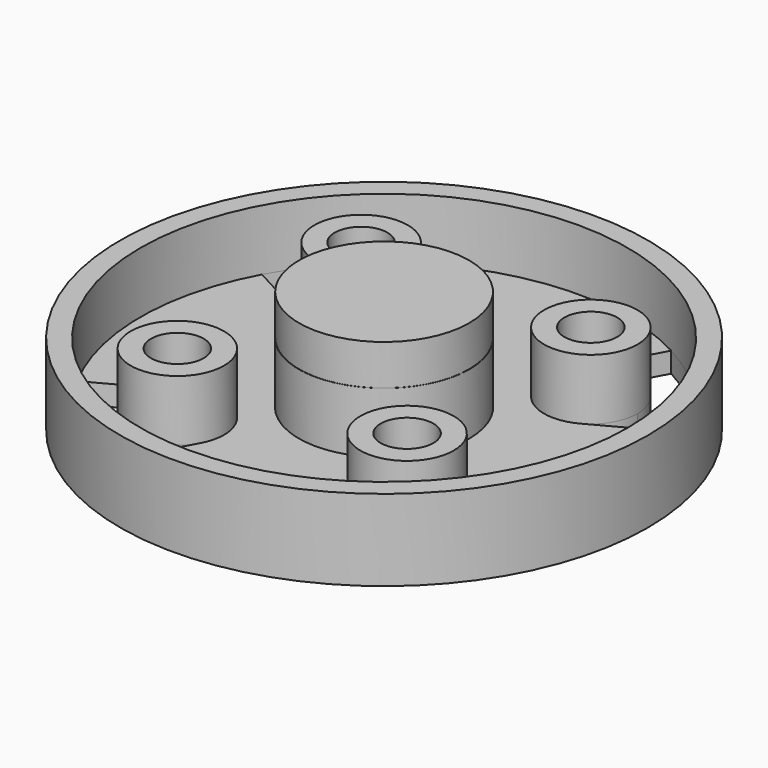
from build123d import *

# Parameters (mm, degrees)
F0_R      = 32.5
F1_DEPTH  = 10
F2_R      = 8
F3_DEPTH  = 25
F4_R      = 3.25
F5_DEPTH  = 25
F6_T      = -2.5
F8_DEPTH  = 25
F9_R      = 10.4716501517
F10_DEPTH = 5


# Not quite as in the source:
# - after a boolean that leaves OpenCascade's solid faulty, fix() repairs it


with BuildPart() as f1:
    # F0 (on Top) → F1 (new body)
    with BuildSketch(Plane.XY):
        Circle(F0_R)
    extrude(amount=F1_DEPTH)

    # F2 (on Top) → F3 (cut)
    with BuildSketch(Plane.XY):
        Circle(F2_R)
    extrude(amount=F3_DEPTH, mode=Mode.SUBTRACT)

    # F4 (on face) → F5 (cut)
    with BuildSketch(Plane.XY.offset(10)):
        with Locations((-14.1421356237, 14.1421356237)):
            Circle(F4_R)
        with Locations((-14.1421356237, -14.1421356237)):
            Circle(F4_R)
        with Locations((14.1421356237, 14.1421356237)):
            Circle(F4_R)
        with Locations((14.1421356237, -14.1421356237)):
            Circle(F4_R)
    extrude(amount=-F5_DEPTH, mode=Mode.SUBTRACT)

    # F6
    f6_openings = [f1.faces().sort_by_distance(p)[0] for p in [
        (-31.580761, 0, 10),
    ]]
    offset(amount=F6_T, openings=f6_openings)

    # F7 (on face) → F8 (cut)
    with BuildSketch(Plane.XY.offset(2.5)):
        with BuildLine():
            ThreePointArc((19.8921356237, 14.1421356237), (19.0783691058, 11.1932207368), (16.8674055331, 9.0789939191))
            Line((16.8674055331, 9.0789939191), (26.4163915025, 14.218799527))
            ThreePointArc((26.4163915025, 14.218799527), (21.2132034356, 21.2132034356), (14.218799527, 26.4163915025))
            Line((14.218799527, 26.4163915025), (9.0789939191, 16.8674055331))
            ThreePointArc((9.0789939191, 16.8674055331), (15.5473820787, 19.7177775061), (19.8921356237, 14.1421356237))
        make_face()
        with BuildLine():
            Line((-9.0789939191, 16.8674055331), (-14.218799527, 26.4163915025))
            ThreePointArc((-14.218799527, 26.4163915025), (-21.2132034356, 21.2132034356), (-26.4163915025, 14.218799527))
            Line((-26.4163915025, 14.218799527), (-16.8674055331, 9.0789939191))
            ThreePointArc((-16.8674055331, 9.0789939191), (-18.2079996156, 18.2079996156), (-9.0789939191, 16.8674055331))
        make_face()
        with BuildLine():
            ThreePointArc((14.218799527, -26.4163915025), (21.2132034356, -21.2132034356), (26.4163915025, -14.218799527))
            Line((26.4163915025, -14.218799527), (16.8674055331, -9.0789939191))
            ThreePointArc((16.8674055331, -9.0789939191), (19.0783691058, -11.1932207368), (19.8921356237, -14.1421356237))
            ThreePointArc((19.8921356237, -14.1421356237), (15.5473820787, -19.7177775061), (9.0789939191, -16.8674055331))
            Line((9.0789939191, -16.8674055331), (14.218799527, -26.4163915025))
        make_face()
        with BuildLine():
            ThreePointArc((-26.4163915025, -14.218799527), (-21.2132034356, -21.2132034356), (-14.218799527, -26.4163915025))
            Line((-14.218799527, -26.4163915025), (-9.0789939191, -16.8674055331))
            ThreePointArc((-9.0789939191, -16.8674055331), (-18.2079996156, -18.2079996156), (-16.8674055331, -9.0789939191))
            Line((-16.8674055331, -9.0789939191), (-26.4163915025, -14.218799527))
        make_face()
    extrude(amount=-F8_DEPTH, mode=Mode.SUBTRACT)

    # F9 (on face) → F10 (join)
    with BuildSketch(Plane.XY.offset(10)):
        Circle(F9_R)
    extrude(amount=F10_DEPTH)

    add(f1.part.fix(), mode=Mode.REPLACE)


solid = f1.part
